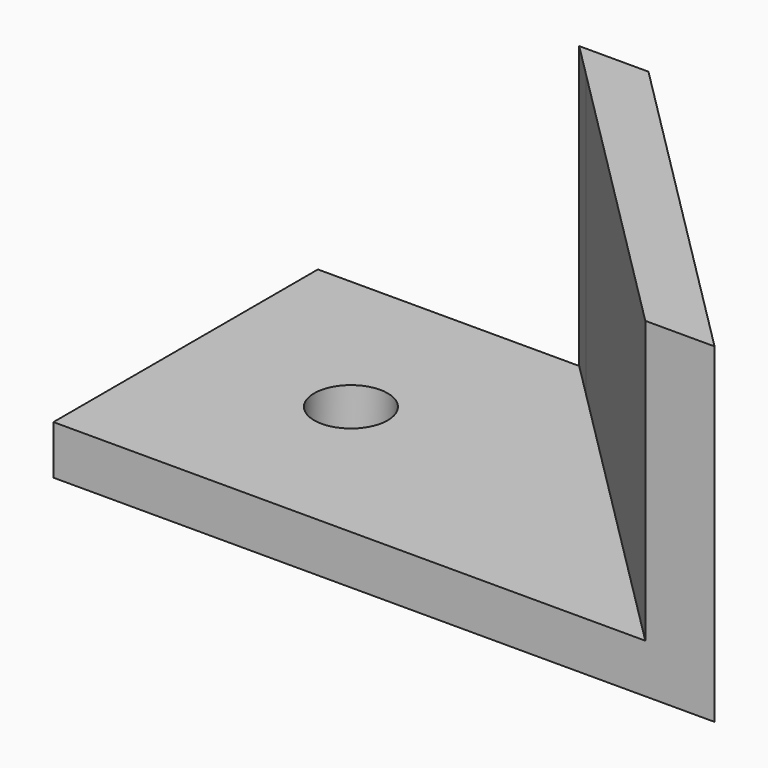
from build123d import *

# Parameters (mm, degrees)
F0_W     = 21.43125
F0_H     = 21.43125
F0_R     = 2.38125
F1_DEPTH = 3.175
F3_DEPTH = 18.25625


# Not quite as in the source:
# - a length typed as a fraction of an inch, garbled in the dataset ("3 / 203.2 mm" for 3/8 in), is restored


with BuildPart() as f1:
    # F0 (on Top) → F1 (new body)
    with BuildSketch(Plane.XY):
        Rectangle(F0_W, F0_H)
        Circle(F0_R, mode=Mode.SUBTRACT)
        Polygon((32.146875, -10.715625), (10.715625, 10.715625), (10.715625, -10.715625), align=None)
    extrude(amount=F1_DEPTH)

    # F2 (on face) → F3 (join)
    with BuildSketch(Plane.XY.offset(3.175)):
        Polygon((32.146875, -10.715625), (10.715625, 10.715625), (8.4705609697, 8.4705609697), (27.6567469395, -10.715625), align=None)
        Polygon((8.4705609697, 8.4705609697), (10.715625, 10.715625), (6.2254969395, 10.715625), align=None)
    extrude(amount=F3_DEPTH)


solid = f1.part
